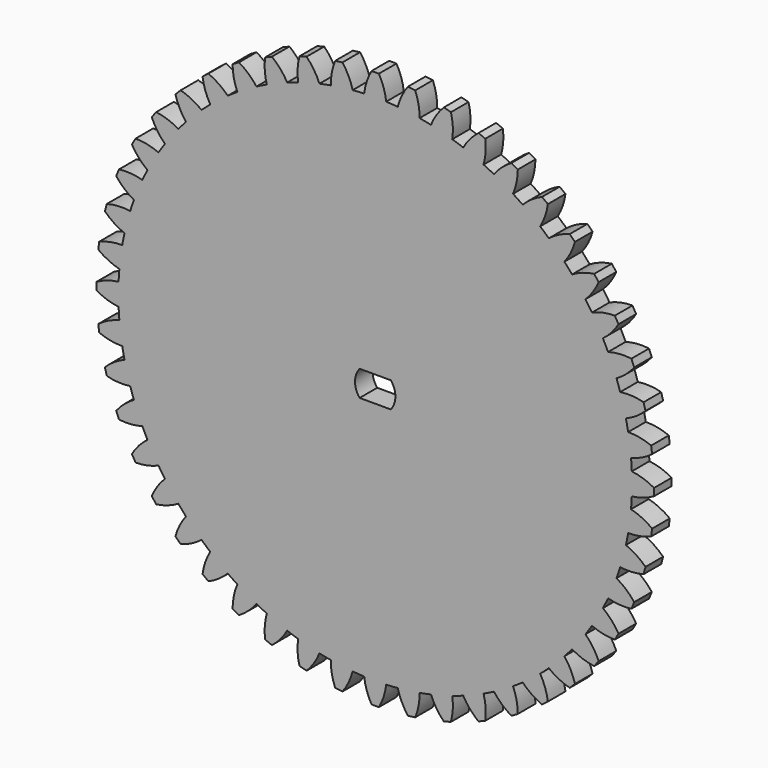
from build123d import *

# Parameters (mm, degrees)
F1_DEPTH = 3


# Not quite as in the source:
# - a feature names something its author has since deleted; it is built from what else it names


with BuildPart() as f1:
    # F0 (on Front) → F1 (new body)
    with BuildSketch(Plane.XZ):
        with BuildLine():
            ThreePointArc((34.9678423698, -1.5), (34.9919596689, -0.7501723324), (35, 0))
            ThreePointArc((35, 0), (34.9919596689, 0.7501723324), (34.9678423698, 1.5))
            ThreePointArc((34.9678423698, 1.5), (34.9250623134, 2.2891095231), (34.8644769192, 3.0770520226))
            ThreePointArc((34.8644769192, 3.0770520226), (34.7005701481, 4.5684167277), (34.4728983425, 6.0513866067))
            ThreePointArc((34.4728983425, 6.0513866067), (34.3274848141, 6.8281612706), (34.1645706023, 7.601454832))
            ThreePointArc((34.1645706023, 7.601454832), (33.8074039201, 9.0586665786), (33.388113467, 10.4992323109))
            ThreePointArc((33.388113467, 10.4992323109), (33.1425545323, 11.2503812856), (32.8800990101, 11.9957946417))
            ThreePointArc((32.8800990101, 11.9957946417), (32.3357836379, 13.3939201328), (31.732048713, 14.7674332392))
            ThreePointArc((31.732048713, 14.7674332392), (31.3905459536, 15.4801041577), (31.0330398078, 16.1848830792))
            ThreePointArc((31.0330398078, 16.1848830792), (30.3108891325, 17.5), (29.5330398078, 18.7829592906))
            ThreePointArc((29.5330398078, 18.7829592906), (29.1014364306, 19.4449581557), (28.6549966904, 20.09704368))
            ThreePointArc((28.6549966904, 20.09704368), (27.7673669102, 21.3066500153), (26.8287124034, 22.4771037008))
            ThreePointArc((26.8287124034, 22.4771037008), (26.3143932618, 23.0771035285), (25.7866586349, 23.6653382914))
            ThreePointArc((25.7866586349, 23.6653382914), (24.7487373415, 24.7487373415), (23.6653382914, 25.7866586349))
            ThreePointArc((23.6653382914, 25.7866586349), (23.0771035285, 26.3143932618), (22.4771037008, 26.8287124034))
            ThreePointArc((22.4771037008, 26.8287124034), (21.3066500153, 27.7673669102), (20.09704368, 28.6549966904))
            ThreePointArc((20.09704368, 28.6549966904), (19.4449581557, 29.1014364306), (18.7829592906, 29.5330398078))
            ThreePointArc((18.7829592906, 29.5330398078), (17.5, 30.3108891325), (16.1848830792, 31.0330398078))
            ThreePointArc((16.1848830792, 31.0330398078), (15.4801041577, 31.3905459536), (14.7674332392, 31.732048713))
            ThreePointArc((14.7674332392, 31.732048713), (13.3939201328, 32.3357836379), (11.9957946417, 32.8800990101))
            ThreePointArc((11.9957946417, 32.8800990101), (11.2503812856, 33.1425545323), (10.4992323109, 33.388113467))
            ThreePointArc((10.4992323109, 33.388113467), (9.0586665786, 33.8074039201), (7.601454832, 34.1645706023))
            ThreePointArc((7.601454832, 34.1645706023), (6.8281612706, 34.3274848141), (6.0513866067, 34.4728983425))
            ThreePointArc((6.0513866067, 34.4728983425), (4.5684167277, 34.7005701481), (3.0770520226, 34.8644769192))
            ThreePointArc((3.0770520226, 34.8644769192), (2.2891095231, 34.9250623134), (1.5, 34.9678423698))
            ThreePointArc((1.5, 34.9678423698), (0, 35), (-1.5, 34.9678423698))
            ThreePointArc((-1.5, 34.9678423698), (-2.2891095231, 34.9250623134), (-3.0770520226, 34.8644769192))
            ThreePointArc((-3.0770520226, 34.8644769192), (-4.5684167277, 34.7005701481), (-6.0513866067, 34.4728983425))
            ThreePointArc((-6.0513866067, 34.4728983425), (-6.8281612706, 34.3274848141), (-7.601454832, 34.1645706023))
            ThreePointArc((-7.601454832, 34.1645706023), (-9.0586665786, 33.8074039201), (-10.4992323109, 33.388113467))
            ThreePointArc((-10.4992323109, 33.388113467), (-11.2503812856, 33.1425545323), (-11.9957946417, 32.8800990101))
            ThreePointArc((-11.9957946417, 32.8800990101), (-13.3939201328, 32.3357836379), (-14.7674332392, 31.732048713))
            ThreePointArc((-14.7674332392, 31.732048713), (-15.4801041577, 31.3905459536), (-16.1848830792, 31.0330398078))
            ThreePointArc((-16.1848830792, 31.0330398078), (-17.5, 30.3108891325), (-18.7829592906, 29.5330398078))
            ThreePointArc((-18.7829592906, 29.5330398078), (-19.4449581557, 29.1014364306), (-20.09704368, 28.6549966904))
            ThreePointArc((-20.09704368, 28.6549966904), (-21.3066500153, 27.7673669102), (-22.4771037008, 26.8287124034))
            ThreePointArc((-22.4771037008, 26.8287124034), (-23.0771035285, 26.3143932618), (-23.6653382914, 25.7866586349))
            ThreePointArc((-23.6653382914, 25.7866586349), (-24.7487373415, 24.7487373415), (-25.7866586349, 23.6653382914))
            ThreePointArc((-25.7866586349, 23.6653382914), (-26.3143932618, 23.0771035285), (-26.8287124034, 22.4771037008))
            ThreePointArc((-26.8287124034, 22.4771037008), (-27.7673669102, 21.3066500153), (-28.6549966904, 20.09704368))
            ThreePointArc((-28.6549966904, 20.09704368), (-29.1014364306, 19.4449581557), (-29.5330398078, 18.7829592906))
            ThreePointArc((-29.5330398078, 18.7829592906), (-30.3108891325, 17.5), (-31.0330398078, 16.1848830792))
            ThreePointArc((-31.0330398078, 16.1848830792), (-31.3905459536, 15.4801041577), (-31.732048713, 14.7674332392))
            ThreePointArc((-31.732048713, 14.7674332392), (-32.3357836379, 13.3939201328), (-32.8800990101, 11.9957946417))
            ThreePointArc((-32.8800990101, 11.9957946417), (-33.1425545323, 11.2503812856), (-33.388113467, 10.4992323109))
            ThreePointArc((-33.388113467, 10.4992323109), (-33.8074039201, 9.0586665786), (-34.1645706023, 7.601454832))
            ThreePointArc((-34.1645706023, 7.601454832), (-34.3274848141, 6.8281612706), (-34.4728983425, 6.0513866067))
            ThreePointArc((-34.4728983425, 6.0513866067), (-34.7005701481, 4.5684167277), (-34.8644769192, 3.0770520226))
            ThreePointArc((-34.8644769192, 3.0770520226), (-34.9250623134, 2.2891095231), (-34.9678423698, 1.5))
            ThreePointArc((-34.9678423698, 1.5), (-35, 0), (-34.9678423698, -1.5))
            ThreePointArc((-34.9678423698, -1.5), (-34.9250623134, -2.2891095231), (-34.8644769192, -3.0770520226))
            ThreePointArc((-34.8644769192, -3.0770520226), (-34.7005701481, -4.5684167277), (-34.4728983425, -6.0513866067))
            ThreePointArc((-34.4728983425, -6.0513866067), (-34.3274848141, -6.8281612706), (-34.1645706023, -7.601454832))
            ThreePointArc((-34.1645706023, -7.601454832), (-33.8074039201, -9.0586665786), (-33.388113467, -10.4992323109))
            ThreePointArc((-33.388113467, -10.4992323109), (-33.1425545323, -11.2503812856), (-32.8800990101, -11.9957946417))
            ThreePointArc((-32.8800990101, -11.9957946417), (-32.3357836379, -13.3939201328), (-31.732048713, -14.7674332392))
            ThreePointArc((-31.732048713, -14.7674332392), (-31.3905459536, -15.4801041577), (-31.0330398078, -16.1848830792))
            ThreePointArc((-31.0330398078, -16.1848830792), (-30.3108891325, -17.5), (-29.5330398078, -18.7829592906))
            ThreePointArc((-29.5330398078, -18.7829592906), (-29.1014364306, -19.4449581557), (-28.6549966904, -20.09704368))
            ThreePointArc((-28.6549966904, -20.09704368), (-27.7673669102, -21.3066500153), (-26.8287124034, -22.4771037008))
            ThreePointArc((-26.8287124034, -22.4771037008), (-26.3143932618, -23.0771035285), (-25.7866586349, -23.6653382914))
            ThreePointArc((-25.7866586349, -23.6653382914), (-24.7487373415, -24.7487373415), (-23.6653382914, -25.7866586349))
            ThreePointArc((-23.6653382914, -25.7866586349), (-23.0771035285, -26.3143932618), (-22.4771037008, -26.8287124034))
            ThreePointArc((-22.4771037008, -26.8287124034), (-21.3066500153, -27.7673669102), (-20.09704368, -28.6549966904))
            ThreePointArc((-20.09704368, -28.6549966904), (-19.4449581557, -29.1014364306), (-18.7829592906, -29.5330398078))
            ThreePointArc((-18.7829592906, -29.5330398078), (-17.5, -30.3108891325), (-16.1848830792, -31.0330398078))
            ThreePointArc((-16.1848830792, -31.0330398078), (-15.4801041577, -31.3905459536), (-14.7674332392, -31.732048713))
            ThreePointArc((-14.7674332392, -31.732048713), (-13.3939201328, -32.3357836379), (-11.9957946417, -32.8800990101))
            ThreePointArc((-11.9957946417, -32.8800990101), (-11.2503812856, -33.1425545323), (-10.4992323109, -33.388113467))
            ThreePointArc((-10.4992323109, -33.388113467), (-9.0586665786, -33.8074039201), (-7.601454832, -34.1645706023))
            ThreePointArc((-7.601454832, -34.1645706023), (-6.8281612706, -34.3274848141), (-6.0513866067, -34.4728983425))
            ThreePointArc((-6.0513866067, -34.4728983425), (-4.5684167277, -34.7005701481), (-3.0770520226, -34.8644769192))
            ThreePointArc((-3.0770520226, -34.8644769192), (-2.2891095231, -34.9250623134), (-1.5, -34.9678423698))
            ThreePointArc((-1.5, -34.9678423698), (0, -35), (1.5, -34.9678423698))
            ThreePointArc((1.5, -34.9678423698), (2.2891095231, -34.9250623134), (3.0770520226, -34.8644769192))
            ThreePointArc((3.0770520226, -34.8644769192), (4.5684167277, -34.7005701481), (6.0513866067, -34.4728983425))
            ThreePointArc((6.0513866067, -34.4728983425), (6.8281612706, -34.3274848141), (7.601454832, -34.1645706023))
            ThreePointArc((7.601454832, -34.1645706023), (9.0586665786, -33.8074039201), (10.4992323109, -33.388113467))
            ThreePointArc((10.4992323109, -33.388113467), (11.2503812856, -33.1425545323), (11.9957946417, -32.8800990101))
            ThreePointArc((11.9957946417, -32.8800990101), (13.3939201328, -32.3357836379), (14.7674332392, -31.732048713))
            ThreePointArc((14.7674332392, -31.732048713), (15.4801041577, -31.3905459536), (16.1848830792, -31.0330398078))
            ThreePointArc((16.1848830792, -31.0330398078), (17.5, -30.3108891325), (18.7829592906, -29.5330398078))
            ThreePointArc((18.7829592906, -29.5330398078), (19.4449581557, -29.1014364306), (20.09704368, -28.6549966904))
            ThreePointArc((20.09704368, -28.6549966904), (21.3066500153, -27.7673669102), (22.4771037008, -26.8287124034))
            ThreePointArc((22.4771037008, -26.8287124034), (23.0771035285, -26.3143932618), (23.6653382914, -25.7866586349))
            ThreePointArc((23.6653382914, -25.7866586349), (24.7487373415, -24.7487373415), (25.7866586349, -23.6653382914))
            ThreePointArc((25.7866586349, -23.6653382914), (26.3143932618, -23.0771035285), (26.8287124034, -22.4771037008))
            ThreePointArc((26.8287124034, -22.4771037008), (27.7673669102, -21.3066500153), (28.6549966904, -20.09704368))
            ThreePointArc((28.6549966904, -20.09704368), (29.1014364306, -19.4449581557), (29.5330398078, -18.7829592906))
            ThreePointArc((29.5330398078, -18.7829592906), (30.3108891325, -17.5), (31.0330398078, -16.1848830792))
            ThreePointArc((31.0330398078, -16.1848830792), (31.3905459536, -15.4801041577), (31.732048713, -14.7674332392))
            ThreePointArc((31.732048713, -14.7674332392), (32.3357836379, -13.3939201328), (32.8800990101, -11.9957946417))
            ThreePointArc((32.8800990101, -11.9957946417), (33.1425545323, -11.2503812856), (33.388113467, -10.4992323109))
            ThreePointArc((33.388113467, -10.4992323109), (33.8074039201, -9.0586665786), (34.1645706023, -7.601454832))
            ThreePointArc((34.1645706023, -7.601454832), (34.3274848141, -6.8281612706), (34.4728983425, -6.0513866067))
            ThreePointArc((34.4728983425, -6.0513866067), (34.7005701481, -4.5684167277), (34.8644769192, -3.0770520226))
            ThreePointArc((34.8644769192, -3.0770520226), (34.9250623134, -2.2891095231), (34.9678423698, -1.5))
        make_face()
        with BuildLine():
            ThreePointArc((2.1213203436, 1.75), (2.5880621075, 0.9297497123), (2.75, 0))
            ThreePointArc((2.75, 0), (2.5880621075, -0.9297497123), (2.1213203436, -1.75))
            ThreePointArc((2.1213203436, -1.75), (0, -2.75), (-2.1213203436, -1.75))
            ThreePointArc((-2.1213203436, -1.75), (-2.75, 0), (-2.1213203436, 1.75))
            ThreePointArc((-2.1213203436, 1.75), (0, 2.75), (2.1213203436, 1.75))
        make_face(mode=Mode.SUBTRACT)
        with BuildLine():
            ThreePointArc((-32.8800990101, 11.9957946417), (-32.3357836379, 13.3939201328), (-31.732048713, 14.7674332392))
            ThreePointArc((-31.732048713, 14.7674332392), (-33.3121475268, 15.0461287529), (-34.9160805192, 15.0039101961))
            Line((-34.9160805192, 15.0039101961), (-35.2987639516, 14.0800306636))
            ThreePointArc((-35.2987639516, 14.0800306636), (-34.1944650839, 12.9160257403), (-32.8800990101, 11.9957946417))
        make_face()
        with BuildLine():
            ThreePointArc((-31.0330398078, 16.1848830792), (-30.3108891325, 17.5), (-29.5330398078, 18.7829592906))
            ThreePointArc((-29.5330398078, 18.7829592906), (-31.063243593, 19.2655148069), (-32.6589653438, 19.4330127019))
            Line((-32.6589653438, 19.4330127019), (-33.1589653438, 18.5669872981))
            ThreePointArc((-33.1589653438, 18.5669872981), (-32.2160470363, 17.268800672), (-31.0330398078, 16.1848830792))
        make_face()
        with BuildLine():
            ThreePointArc((-28.6549966904, 20.09704368), (-27.7673669102, 21.3066500153), (-26.8287124034, 22.4771037008))
            ThreePointArc((-26.8287124034, 22.4771037008), (-28.282838949, 23.1552625613), (-29.8430462166, 23.5296109725))
            Line((-29.8430462166, 23.5296109725), (-30.4518076456, 22.7362576322))
            ThreePointArc((-30.4518076456, 22.7362576322), (-29.686403492, 21.3261016364), (-28.6549966904, 20.09704368))
        make_face()
        with BuildLine():
            ThreePointArc((-25.7866586349, 23.6653382914), (-24.7487373415, 24.7487373415), (-23.6653382914, 25.7866586349))
            ThreePointArc((-23.6653382914, 25.7866586349), (-25.0185070891, 26.6488173533), (-26.5165042945, 27.2236110757))
            Line((-26.5165042945, 27.2236110757), (-27.2236110757, 26.5165042945))
            ThreePointArc((-27.2236110757, 26.5165042945), (-26.6488173533, 25.0185070891), (-25.7866586349, 23.6653382914))
        make_face()
        with BuildLine():
            ThreePointArc((-22.4771037008, 26.8287124034), (-21.3066500153, 27.7673669102), (-20.09704368, 28.6549966904))
            ThreePointArc((-20.09704368, 28.6549966904), (-21.3261016364, 29.686403492), (-22.7362576322, 30.4518076456))
            Line((-22.7362576322, 30.4518076456), (-23.5296109725, 29.8430462166))
            ThreePointArc((-23.5296109725, 29.8430462166), (-23.1552625613, 28.282838949), (-22.4771037008, 26.8287124034))
        make_face()
        with BuildLine():
            ThreePointArc((-18.7829592906, 29.5330398078), (-17.5, 30.3108891325), (-16.1848830792, 31.0330398078))
            ThreePointArc((-16.1848830792, 31.0330398078), (-17.268800672, 32.2160470363), (-18.5669872981, 33.1589653438))
            Line((-18.5669872981, 33.1589653438), (-19.4330127019, 32.6589653438))
            ThreePointArc((-19.4330127019, 32.6589653438), (-19.2655148069, 31.063243593), (-18.7829592906, 29.5330398078))
        make_face()
        with BuildLine():
            ThreePointArc((-6.0513866067, 34.4728983425), (-4.5684167277, 34.7005701481), (-3.0770520226, 34.8644769192))
            ThreePointArc((-3.0770520226, 34.8644769192), (-3.6257440348, 36.3722303893), (-4.4642728737, 37.7401678283))
            Line((-4.4642728737, 37.7401678283), (-5.455717735, 37.6096416361))
            ThreePointArc((-5.455717735, 37.6096416361), (-5.9116261349, 36.0712883016), (-6.0513866067, 34.4728983425))
        make_face()
        with BuildLine():
            ThreePointArc((-1.5, 34.9678423698), (0, 35), (1.5, 34.9678423698))
            ThreePointArc((1.5, 34.9678423698), (1.1528034433, 36.534315479), (0.5, 38))
            Line((0.5, 38), (-0.5, 38))
            ThreePointArc((-0.5, 38), (-1.1528034433, 36.534315479), (-1.5, 34.9678423698))
        make_face()
        with BuildLine():
            ThreePointArc((-10.4992323109, 33.388113467), (-9.0586665786, 33.8074039201), (-7.601454832, 34.1645706023))
            ThreePointArc((-7.601454832, 34.1645706023), (-8.3422540272, 35.5878063533), (-9.3521608008, 36.8345909215))
            Line((-9.3521608008, 36.8345909215), (-10.318086627, 36.5757718764))
            ThreePointArc((-10.318086627, 36.5757718764), (-10.5692992642, 34.9910713806), (-10.4992323109, 33.388113467))
        make_face()
        with BuildLine():
            ThreePointArc((-14.7674332392, 31.732048713), (-13.3939201328, 32.3357836379), (-11.9957946417, 32.8800990101))
            ThreePointArc((-11.9957946417, 32.8800990101), (-12.9160257403, 34.1944650839), (-14.0800306636, 35.2987639516))
            Line((-14.0800306636, 35.2987639516), (-15.0039101961, 34.9160805192))
            ThreePointArc((-15.0039101961, 34.9160805192), (-15.0461287529, 33.3121475268), (-14.7674332392, 31.732048713))
        make_face()
        with BuildLine():
            ThreePointArc((3.0770520226, 34.8644769192), (4.5684167277, 34.7005701481), (6.0513866067, 34.4728983425))
            ThreePointArc((6.0513866067, 34.4728983425), (5.9116261349, 36.0712883016), (5.455717735, 37.6096416361))
            Line((5.455717735, 37.6096416361), (4.4642728737, 37.7401678283))
            ThreePointArc((4.4642728737, 37.7401678283), (3.6257440348, 36.3722303893), (3.0770520226, 34.8644769192))
        make_face()
        with BuildLine():
            ThreePointArc((7.601454832, 34.1645706023), (9.0586665786, 33.8074039201), (10.4992323109, 33.388113467))
            ThreePointArc((10.4992323109, 33.388113467), (10.5692992642, 34.9910713806), (10.318086627, 36.5757718764))
            Line((10.318086627, 36.5757718764), (9.3521608008, 36.8345909215))
            ThreePointArc((9.3521608008, 36.8345909215), (8.3422540272, 35.5878063533), (7.601454832, 34.1645706023))
        make_face()
        with BuildLine():
            ThreePointArc((11.9957946417, 32.8800990101), (13.3939201328, 32.3357836379), (14.7674332392, 31.732048713))
            ThreePointArc((14.7674332392, 31.732048713), (15.0461287529, 33.3121475268), (15.0039101961, 34.9160805192))
            Line((15.0039101961, 34.9160805192), (14.0800306636, 35.2987639516))
            ThreePointArc((14.0800306636, 35.2987639516), (12.9160257403, 34.1944650839), (11.9957946417, 32.8800990101))
        make_face()
        with BuildLine():
            ThreePointArc((16.1848830792, 31.0330398078), (17.5, 30.3108891325), (18.7829592906, 29.5330398078))
            ThreePointArc((18.7829592906, 29.5330398078), (19.2655148069, 31.063243593), (19.4330127019, 32.6589653438))
            Line((19.4330127019, 32.6589653438), (18.5669872981, 33.1589653438))
            ThreePointArc((18.5669872981, 33.1589653438), (17.268800672, 32.2160470363), (16.1848830792, 31.0330398078))
        make_face()
        with BuildLine():
            ThreePointArc((20.09704368, 28.6549966904), (21.3066500153, 27.7673669102), (22.4771037008, 26.8287124034))
            ThreePointArc((22.4771037008, 26.8287124034), (23.1552625613, 28.282838949), (23.5296109725, 29.8430462166))
            Line((23.5296109725, 29.8430462166), (22.7362576322, 30.4518076456))
            ThreePointArc((22.7362576322, 30.4518076456), (21.3261016364, 29.686403492), (20.09704368, 28.6549966904))
        make_face()
        with BuildLine():
            ThreePointArc((23.6653382914, 25.7866586349), (24.7487373415, 24.7487373415), (25.7866586349, 23.6653382914))
            ThreePointArc((25.7866586349, 23.6653382914), (26.6488173533, 25.0185070891), (27.2236110757, 26.5165042945))
            Line((27.2236110757, 26.5165042945), (26.5165042945, 27.2236110757))
            ThreePointArc((26.5165042945, 27.2236110757), (25.0185070891, 26.6488173533), (23.6653382914, 25.7866586349))
        make_face()
        with BuildLine():
            ThreePointArc((26.8287124034, 22.4771037008), (27.7673669102, 21.3066500153), (28.6549966904, 20.09704368))
            ThreePointArc((28.6549966904, 20.09704368), (29.686403492, 21.3261016364), (30.4518076456, 22.7362576322))
            Line((30.4518076456, 22.7362576322), (29.8430462166, 23.5296109725))
            ThreePointArc((29.8430462166, 23.5296109725), (28.282838949, 23.1552625613), (26.8287124034, 22.4771037008))
        make_face()
        with BuildLine():
            ThreePointArc((29.5330398078, 18.7829592906), (30.3108891325, 17.5), (31.0330398078, 16.1848830792))
            ThreePointArc((31.0330398078, 16.1848830792), (32.2160470363, 17.268800672), (33.1589653438, 18.5669872981))
            Line((33.1589653438, 18.5669872981), (32.6589653438, 19.4330127019))
            ThreePointArc((32.6589653438, 19.4330127019), (31.063243593, 19.2655148069), (29.5330398078, 18.7829592906))
        make_face()
        with BuildLine():
            ThreePointArc((31.732048713, 14.7674332392), (32.3357836379, 13.3939201328), (32.8800990101, 11.9957946417))
            ThreePointArc((32.8800990101, 11.9957946417), (34.1944650839, 12.9160257403), (35.2987639516, 14.0800306636))
            Line((35.2987639516, 14.0800306636), (34.9160805192, 15.0039101961))
            ThreePointArc((34.9160805192, 15.0039101961), (33.3121475268, 15.0461287529), (31.732048713, 14.7674332392))
        make_face()
        with BuildLine():
            ThreePointArc((33.388113467, 10.4992323109), (33.8074039201, 9.0586665786), (34.1645706023, 7.601454832))
            ThreePointArc((34.1645706023, 7.601454832), (35.5878063533, 8.3422540272), (36.8345909215, 9.3521608008))
            Line((36.8345909215, 9.3521608008), (36.5757718764, 10.318086627))
            ThreePointArc((36.5757718764, 10.318086627), (34.9910713806, 10.5692992642), (33.388113467, 10.4992323109))
        make_face()
        with BuildLine():
            ThreePointArc((34.4728983425, 6.0513866067), (34.7005701481, 4.5684167277), (34.8644769192, 3.0770520226))
            ThreePointArc((34.8644769192, 3.0770520226), (36.3722303893, 3.6257440348), (37.7401678283, 4.4642728737))
            Line((37.7401678283, 4.4642728737), (37.6096416361, 5.455717735))
            ThreePointArc((37.6096416361, 5.455717735), (36.0712883016, 5.9116261349), (34.4728983425, 6.0513866067))
        make_face()
        with BuildLine():
            ThreePointArc((34.9678423698, 1.5), (34.9919596689, 0.7501723324), (35, 0))
            ThreePointArc((35, 0), (34.9919596689, -0.7501723324), (34.9678423698, -1.5))
            ThreePointArc((34.9678423698, -1.5), (36.534315479, -1.1528034433), (38, -0.5))
            Line((38, -0.5), (38, 0.5))
            ThreePointArc((38, 0.5), (36.534315479, 1.1528034433), (34.9678423698, 1.5))
        make_face()
        with BuildLine():
            ThreePointArc((37.7401678283, -4.4642728737), (36.3722303893, -3.6257440348), (34.8644769192, -3.0770520226))
            ThreePointArc((34.8644769192, -3.0770520226), (34.7005701481, -4.5684167277), (34.4728983425, -6.0513866067))
            ThreePointArc((34.4728983425, -6.0513866067), (36.0712883016, -5.9116261349), (37.6096416361, -5.455717735))
            Line((37.6096416361, -5.455717735), (37.7401678283, -4.4642728737))
        make_face()
        with BuildLine():
            ThreePointArc((36.8345909215, -9.3521608008), (35.5878063533, -8.3422540272), (34.1645706023, -7.601454832))
            ThreePointArc((34.1645706023, -7.601454832), (33.8074039201, -9.0586665786), (33.388113467, -10.4992323109))
            ThreePointArc((33.388113467, -10.4992323109), (34.9910713806, -10.5692992642), (36.5757718764, -10.318086627))
            Line((36.5757718764, -10.318086627), (36.8345909215, -9.3521608008))
        make_face()
        with BuildLine():
            ThreePointArc((35.2987639516, -14.0800306636), (34.1944650839, -12.9160257403), (32.8800990101, -11.9957946417))
            ThreePointArc((32.8800990101, -11.9957946417), (32.3357836379, -13.3939201328), (31.732048713, -14.7674332392))
            ThreePointArc((31.732048713, -14.7674332392), (33.3121475268, -15.0461287529), (34.9160805192, -15.0039101961))
            Line((34.9160805192, -15.0039101961), (35.2987639516, -14.0800306636))
        make_face()
        with BuildLine():
            ThreePointArc((33.1589653438, -18.5669872981), (32.2160470363, -17.268800672), (31.0330398078, -16.1848830792))
            ThreePointArc((31.0330398078, -16.1848830792), (30.3108891325, -17.5), (29.5330398078, -18.7829592906))
            ThreePointArc((29.5330398078, -18.7829592906), (31.063243593, -19.2655148069), (32.6589653438, -19.4330127019))
            Line((32.6589653438, -19.4330127019), (33.1589653438, -18.5669872981))
        make_face()
        with BuildLine():
            ThreePointArc((30.4518076456, -22.7362576322), (29.686403492, -21.3261016364), (28.6549966904, -20.09704368))
            ThreePointArc((28.6549966904, -20.09704368), (27.7673669102, -21.3066500153), (26.8287124034, -22.4771037008))
            ThreePointArc((26.8287124034, -22.4771037008), (28.282838949, -23.1552625613), (29.8430462166, -23.5296109725))
            Line((29.8430462166, -23.5296109725), (30.4518076456, -22.7362576322))
        make_face()
        with BuildLine():
            ThreePointArc((27.2236110757, -26.5165042945), (26.6488173533, -25.0185070891), (25.7866586349, -23.6653382914))
            ThreePointArc((25.7866586349, -23.6653382914), (24.7487373415, -24.7487373415), (23.6653382914, -25.7866586349))
            ThreePointArc((23.6653382914, -25.7866586349), (25.0185070891, -26.6488173533), (26.5165042945, -27.2236110757))
            Line((26.5165042945, -27.2236110757), (27.2236110757, -26.5165042945))
        make_face()
        with BuildLine():
            ThreePointArc((23.5296109725, -29.8430462166), (23.1552625613, -28.282838949), (22.4771037008, -26.8287124034))
            ThreePointArc((22.4771037008, -26.8287124034), (21.3066500153, -27.7673669102), (20.09704368, -28.6549966904))
            ThreePointArc((20.09704368, -28.6549966904), (21.3261016364, -29.686403492), (22.7362576322, -30.4518076456))
            Line((22.7362576322, -30.4518076456), (23.5296109725, -29.8430462166))
        make_face()
        with BuildLine():
            ThreePointArc((19.4330127019, -32.6589653438), (19.2655148069, -31.063243593), (18.7829592906, -29.5330398078))
            ThreePointArc((18.7829592906, -29.5330398078), (17.5, -30.3108891325), (16.1848830792, -31.0330398078))
            ThreePointArc((16.1848830792, -31.0330398078), (17.268800672, -32.2160470363), (18.5669872981, -33.1589653438))
            Line((18.5669872981, -33.1589653438), (19.4330127019, -32.6589653438))
        make_face()
        with BuildLine():
            ThreePointArc((15.0039101961, -34.9160805192), (15.0461287529, -33.3121475268), (14.7674332392, -31.732048713))
            ThreePointArc((14.7674332392, -31.732048713), (13.3939201328, -32.3357836379), (11.9957946417, -32.8800990101))
            ThreePointArc((11.9957946417, -32.8800990101), (12.9160257403, -34.1944650839), (14.0800306636, -35.2987639516))
            Line((14.0800306636, -35.2987639516), (15.0039101961, -34.9160805192))
        make_face()
        with BuildLine():
            ThreePointArc((10.318086627, -36.5757718764), (10.5692992642, -34.9910713806), (10.4992323109, -33.388113467))
            ThreePointArc((10.4992323109, -33.388113467), (9.0586665786, -33.8074039201), (7.601454832, -34.1645706023))
            ThreePointArc((7.601454832, -34.1645706023), (8.3422540272, -35.5878063533), (9.3521608008, -36.8345909215))
            Line((9.3521608008, -36.8345909215), (10.318086627, -36.5757718764))
        make_face()
        with BuildLine():
            ThreePointArc((5.455717735, -37.6096416361), (5.9116261349, -36.0712883016), (6.0513866067, -34.4728983425))
            ThreePointArc((6.0513866067, -34.4728983425), (4.5684167277, -34.7005701481), (3.0770520226, -34.8644769192))
            ThreePointArc((3.0770520226, -34.8644769192), (3.6257440348, -36.3722303893), (4.4642728737, -37.7401678283))
            Line((4.4642728737, -37.7401678283), (5.455717735, -37.6096416361))
        make_face()
        with BuildLine():
            ThreePointArc((0.5, -38), (1.1528034433, -36.534315479), (1.5, -34.9678423698))
            ThreePointArc((1.5, -34.9678423698), (0, -35), (-1.5, -34.9678423698))
            ThreePointArc((-1.5, -34.9678423698), (-1.1528034433, -36.534315479), (-0.5, -38))
            Line((-0.5, -38), (0.5, -38))
        make_face()
        with BuildLine():
            ThreePointArc((-4.4642728737, -37.7401678283), (-3.6257440348, -36.3722303893), (-3.0770520226, -34.8644769192))
            ThreePointArc((-3.0770520226, -34.8644769192), (-4.5684167277, -34.7005701481), (-6.0513866067, -34.4728983425))
            ThreePointArc((-6.0513866067, -34.4728983425), (-5.9116261349, -36.0712883016), (-5.455717735, -37.6096416361))
            Line((-5.455717735, -37.6096416361), (-4.4642728737, -37.7401678283))
        make_face()
        with BuildLine():
            ThreePointArc((-9.3521608008, -36.8345909215), (-8.3422540272, -35.5878063533), (-7.601454832, -34.1645706023))
            ThreePointArc((-7.601454832, -34.1645706023), (-9.0586665786, -33.8074039201), (-10.4992323109, -33.388113467))
            ThreePointArc((-10.4992323109, -33.388113467), (-10.5692992642, -34.9910713806), (-10.318086627, -36.5757718764))
            Line((-10.318086627, -36.5757718764), (-9.3521608008, -36.8345909215))
        make_face()
        with BuildLine():
            ThreePointArc((-14.0800306636, -35.2987639516), (-12.9160257403, -34.1944650839), (-11.9957946417, -32.8800990101))
            ThreePointArc((-11.9957946417, -32.8800990101), (-13.3939201328, -32.3357836379), (-14.7674332392, -31.732048713))
            ThreePointArc((-14.7674332392, -31.732048713), (-15.0461287529, -33.3121475268), (-15.0039101961, -34.9160805192))
            Line((-15.0039101961, -34.9160805192), (-14.0800306636, -35.2987639516))
        make_face()
        with BuildLine():
            ThreePointArc((-18.5669872981, -33.1589653438), (-17.268800672, -32.2160470363), (-16.1848830792, -31.0330398078))
            ThreePointArc((-16.1848830792, -31.0330398078), (-17.5, -30.3108891325), (-18.7829592906, -29.5330398078))
            ThreePointArc((-18.7829592906, -29.5330398078), (-19.2655148069, -31.063243593), (-19.4330127019, -32.6589653438))
            Line((-19.4330127019, -32.6589653438), (-18.5669872981, -33.1589653438))
        make_face()
        with BuildLine():
            ThreePointArc((-22.7362576322, -30.4518076456), (-21.3261016364, -29.686403492), (-20.09704368, -28.6549966904))
            ThreePointArc((-20.09704368, -28.6549966904), (-21.3066500153, -27.7673669102), (-22.4771037008, -26.8287124034))
            ThreePointArc((-22.4771037008, -26.8287124034), (-23.1552625613, -28.282838949), (-23.5296109725, -29.8430462166))
            Line((-23.5296109725, -29.8430462166), (-22.7362576322, -30.4518076456))
        make_face()
        with BuildLine():
            ThreePointArc((-26.5165042945, -27.2236110757), (-25.0185070891, -26.6488173533), (-23.6653382914, -25.7866586349))
            ThreePointArc((-23.6653382914, -25.7866586349), (-24.7487373415, -24.7487373415), (-25.7866586349, -23.6653382914))
            ThreePointArc((-25.7866586349, -23.6653382914), (-26.6488173533, -25.0185070891), (-27.2236110757, -26.5165042945))
            Line((-27.2236110757, -26.5165042945), (-26.5165042945, -27.2236110757))
        make_face()
        with BuildLine():
            ThreePointArc((-29.8430462166, -23.5296109725), (-28.282838949, -23.1552625613), (-26.8287124034, -22.4771037008))
            ThreePointArc((-26.8287124034, -22.4771037008), (-27.7673669102, -21.3066500153), (-28.6549966904, -20.09704368))
            ThreePointArc((-28.6549966904, -20.09704368), (-29.686403492, -21.3261016364), (-30.4518076456, -22.7362576322))
            Line((-30.4518076456, -22.7362576322), (-29.8430462166, -23.5296109725))
        make_face()
        with BuildLine():
            ThreePointArc((-32.6589653438, -19.4330127019), (-31.063243593, -19.2655148069), (-29.5330398078, -18.7829592906))
            ThreePointArc((-29.5330398078, -18.7829592906), (-30.3108891325, -17.5), (-31.0330398078, -16.1848830792))
            ThreePointArc((-31.0330398078, -16.1848830792), (-32.2160470363, -17.268800672), (-33.1589653438, -18.5669872981))
            Line((-33.1589653438, -18.5669872981), (-32.6589653438, -19.4330127019))
        make_face()
        with BuildLine():
            ThreePointArc((-34.9160805192, -15.0039101961), (-33.3121475268, -15.0461287529), (-31.732048713, -14.7674332392))
            ThreePointArc((-31.732048713, -14.7674332392), (-32.3357836379, -13.3939201328), (-32.8800990101, -11.9957946417))
            ThreePointArc((-32.8800990101, -11.9957946417), (-34.1944650839, -12.9160257403), (-35.2987639516, -14.0800306636))
            Line((-35.2987639516, -14.0800306636), (-34.9160805192, -15.0039101961))
        make_face()
        with BuildLine():
            ThreePointArc((-36.5757718764, -10.318086627), (-34.9910713806, -10.5692992642), (-33.388113467, -10.4992323109))
            ThreePointArc((-33.388113467, -10.4992323109), (-33.8074039201, -9.0586665786), (-34.1645706023, -7.601454832))
            ThreePointArc((-34.1645706023, -7.601454832), (-35.5878063533, -8.3422540272), (-36.8345909215, -9.3521608008))
            Line((-36.8345909215, -9.3521608008), (-36.5757718764, -10.318086627))
        make_face()
        with BuildLine():
            ThreePointArc((-37.6096416361, -5.455717735), (-36.0712883016, -5.9116261349), (-34.4728983425, -6.0513866067))
            ThreePointArc((-34.4728983425, -6.0513866067), (-34.7005701481, -4.5684167277), (-34.8644769192, -3.0770520226))
            ThreePointArc((-34.8644769192, -3.0770520226), (-36.3722303893, -3.6257440348), (-37.7401678283, -4.4642728737))
            Line((-37.7401678283, -4.4642728737), (-37.6096416361, -5.455717735))
        make_face()
        with BuildLine():
            ThreePointArc((-34.9678423698, -1.5), (-35, 0), (-34.9678423698, 1.5))
            ThreePointArc((-34.9678423698, 1.5), (-36.534315479, 1.1528034433), (-38, 0.5))
            Line((-38, 0.5), (-38, -0.5))
            ThreePointArc((-38, -0.5), (-36.534315479, -1.1528034433), (-34.9678423698, -1.5))
        make_face()
        with BuildLine():
            ThreePointArc((-34.8644769192, 3.0770520226), (-34.7005701481, 4.5684167277), (-34.4728983425, 6.0513866067))
            ThreePointArc((-34.4728983425, 6.0513866067), (-36.0712883016, 5.9116261349), (-37.6096416361, 5.455717735))
            Line((-37.6096416361, 5.455717735), (-37.7401678283, 4.4642728737))
            ThreePointArc((-37.7401678283, 4.4642728737), (-36.3722303893, 3.6257440348), (-34.8644769192, 3.0770520226))
        make_face()
        with BuildLine():
            ThreePointArc((-34.1645706023, 7.601454832), (-33.8074039201, 9.0586665786), (-33.388113467, 10.4992323109))
            ThreePointArc((-33.388113467, 10.4992323109), (-34.9910713806, 10.5692992642), (-36.5757718764, 10.318086627))
            Line((-36.5757718764, 10.318086627), (-36.8345909215, 9.3521608008))
            ThreePointArc((-36.8345909215, 9.3521608008), (-35.5878063533, 8.3422540272), (-34.1645706023, 7.601454832))
        make_face()
        with BuildLine():
            Line((-2.1213203436, 1.75), (2.1213203436, 1.75))
            ThreePointArc((2.1213203436, 1.75), (0, 2.75), (-2.1213203436, 1.75))
        make_face()
        with BuildLine():
            ThreePointArc((-2.1213203436, -1.75), (0, -2.75), (2.1213203436, -1.75))
            Line((2.1213203436, -1.75), (-2.1213203436, -1.75))
        make_face()
    extrude(amount=F1_DEPTH)


solid = f1.part
